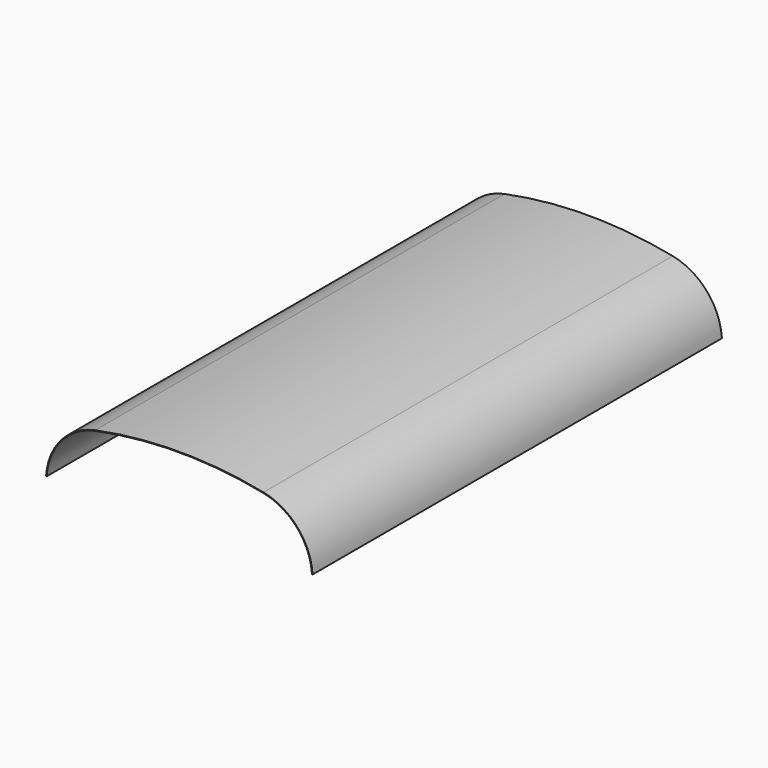
from build123d import *

# Parameters (mm, degrees)
F1_DEPTH = 2526


with BuildPart() as f1:
    # F0 (on Front) → F1 (new body)
    with BuildSketch(Plane.XZ):
        with BuildLine():
            ThreePointArc((-414.6836784295, 1458.609211018), (0, 1500), (414.6836784295, 1458.609211018))
            ThreePointArc((414.6836784295, 1458.609211018), (581.5981876067, 1361.576932454), (654.8216297668, 1182.9319102019))
            Line((654.8216297668, 1182.9319102019), (657.8159792684, 1183.1159511275))
            ThreePointArc((657.8159792684, 1183.1159511275), (583.8603026867, 1363.5474236021), (415.2766484177, 1461.5500249518))
            ThreePointArc((415.2766484177, 1461.5500249518), (0, 1503), (-415.2766484177, 1461.5500249518))
            ThreePointArc((-415.2766484177, 1461.5500249518), (-583.8603026867, 1363.5474236021), (-657.8159792684, 1183.1159511275))
            Line((-657.8159792684, 1183.1159511275), (-654.8216297668, 1182.9319102019))
            ThreePointArc((-654.8216297668, 1182.9319102019), (-581.5981876067, 1361.576932454), (-414.6836784295, 1458.609211018))
        make_face()
    extrude(amount=F1_DEPTH)


solid = f1.part
